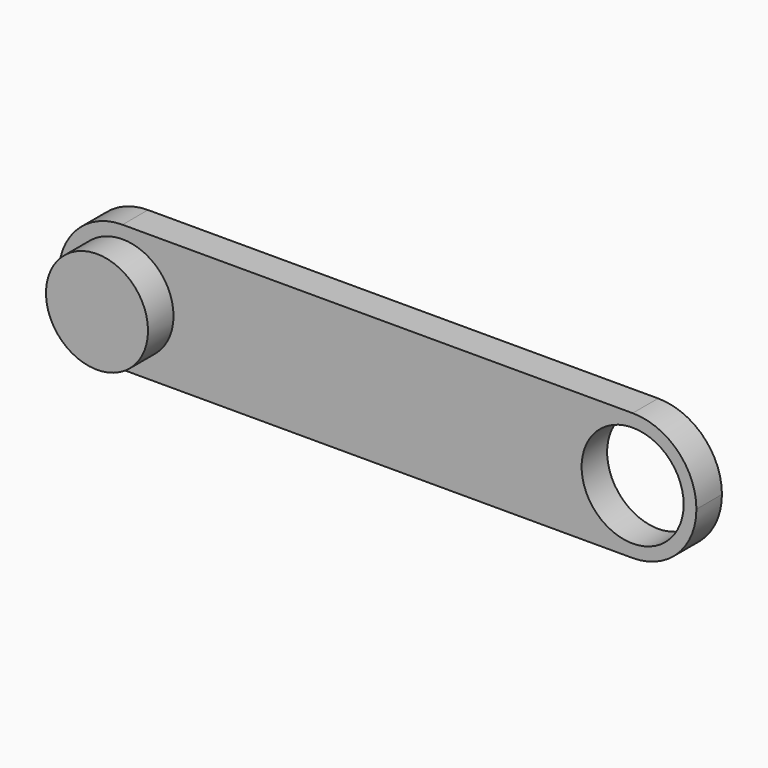
from build123d import *

# Parameters (mm, degrees)
F2_DEPTH = 12.7
F3_R     = 20.32
F4_DEPTH = 12.7
F5_DEPTH = 12.7


# Not quite as in the source:
# - a variable given as a bare number and used for a length is read in inches; the dataset says mm whatever the document's units were


with BuildPart() as f2:
    # F1 (on Front) → F2 (new body)
    with BuildSketch(Plane.XZ):
        with BuildLine():
            Line((152.3496784632, 52.2385248174), (-50.8503215368, 52.2385248174))
            ThreePointArc((-50.8503215368, 52.2385248174), (-68.8108337789, 44.7990370595), (-76.2503215368, 26.8385248174))
            ThreePointArc((-76.2503215368, 26.8385248174), (-68.8108337789, 8.8780125752), (-50.8503215368, 1.4385248174))
            Line((-50.8503215368, 1.4385248174), (152.3496784632, 1.4385248174))
            ThreePointArc((152.3496784632, 1.4385248174), (170.3101907054, 8.8780125752), (177.7496784632, 26.8385248174))
            ThreePointArc((177.7496784632, 26.8385248174), (170.3101907054, 44.7990370595), (152.3496784632, 52.2385248174))
        make_face()
    extrude(amount=F2_DEPTH)

    # F3 (on face) → F4 (join)
    with BuildSketch(Plane.XZ.offset(12.7)):
        with Locations((-50.8503215368, 26.8385248174)):
            Circle(F3_R)
    extrude(amount=F4_DEPTH)

    # F3 (on face) → F5 (cut)
    with BuildSketch(Plane.XZ.offset(12.7)):
        with Locations((152.3496784632, 26.8385248174)):
            Circle(F3_R)
    extrude(amount=-F5_DEPTH, mode=Mode.SUBTRACT)


solid = f2.part
